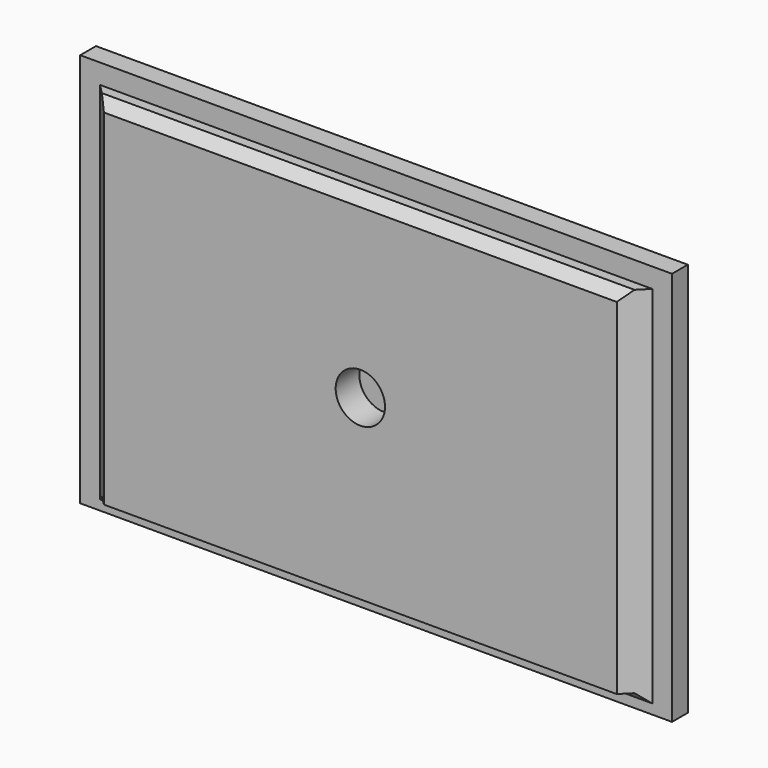
from build123d import *

# Parameters (mm, degrees)
F0_W          = 300
F0_H          = 200
F1_DEPTH      = 10
F2_W          = 280
F2_H          = 180
F3_DEPTH      = 10
F4_SIZE       = 5
F5_SIZE       = 9.99999
F6_R          = 12.5
F7_DEPTH      = 15
F8_W          = 290
F8_H          = 190
F9_DEPTH      = 3
F10_TEXT_SIZE = 58.0489741794
F11_DEPTH     = 5


# Not quite as in the source:
# - a fillet or chamfer is up to 0.001 mm smaller than in the source, because OpenCascade refuses the exact size
# - Text() gives the source's letters only with a copy of the font that has no kerning and outlines rounded to 1/6400 em; it was checked with that copy


with BuildPart() as f1:
    # F0 (on Front) → F1 (new body)
    with BuildSketch(Plane.XZ):
        Rectangle(F0_W, F0_H)
    extrude(amount=F1_DEPTH)

    # F2 (on face) → F3 (join)
    with BuildSketch(Plane.XZ.offset(10)):
        Rectangle(F2_W, F2_H)
    extrude(amount=F3_DEPTH)

    # F4
    f4_edges = [f1.edges().sort_by_distance(p)[0] for p in [
        (0, -20, 90),
        (0, -10, -90),
    ]]
    chamfer(f4_edges, length=F4_SIZE)

    # F5 (size 10 in the source; OpenCascade refuses exactly that, so slightly less here)
    f5_edges = [f1.edges().sort_by_distance(p)[0] for p in [
        (-140, -20, -2.5),
        (140, -20, -2.5),
    ]]
    chamfer(f5_edges, length=F5_SIZE)

    # F6 (on face) → F7 (cut)
    with BuildSketch(Plane.XZ.offset(20)):
        Circle(F6_R)
    extrude(amount=-F7_DEPTH, mode=Mode.SUBTRACT)

    # F8 (on face) → F9 (cut)
    with BuildSketch(Plane(origin=(0, 0, 0), x_dir=(-1, 0, 0), z_dir=(0, 1, 0))):
        Rectangle(F8_W, F8_H)
    extrude(amount=-F9_DEPTH, mode=Mode.SUBTRACT)

    # F10 (on face) → F11 (join)
    with BuildSketch(Plane(origin=(0, -3, 0), x_dir=(-1, 0, 0), z_dir=(0, 1, 0))):
        with Locations((0, -76.6871107396)):
            Text('LJH', F10_TEXT_SIZE, font='Open Sans', text_align=(TextAlign.LEFT, TextAlign.BOTTOM))
    extrude(amount=F11_DEPTH)


solid = f1.part
